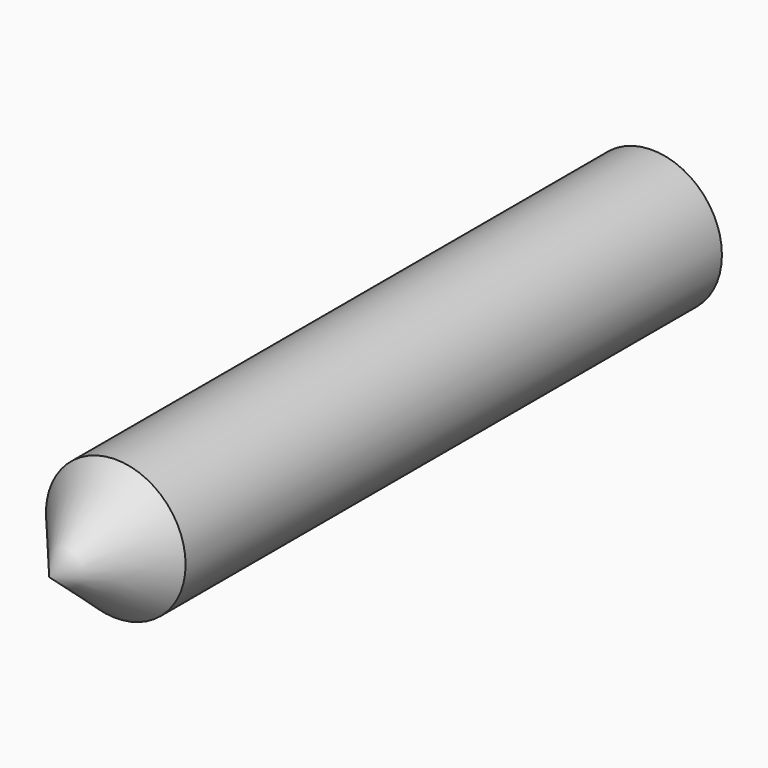
from build123d import *

# Parameters (mm, degrees)
F0_R     = 15.875
F0_R_2   = 12.7
F1_DEPTH = 152.4
F2_R     = 15.875


# Not quite as in the source:
# - an extrude whose draft closes it to a point is written as a loft to that point


with BuildPart() as f1:
    # F0 (on Front) → F1 (new body)
    with BuildSketch(Plane.XZ):
        Circle(F0_R)
        Circle(F0_R_2, mode=Mode.SUBTRACT)
    extrude(amount=F1_DEPTH)

    # F2 (on face) → F3 section 0
    with BuildSketch(Plane.XZ.offset(152.4), mode=Mode.PRIVATE) as f3_s0:
        Circle(F2_R)
    loft([f3_s0.sketch, Vertex(0, -171.3190882824, 0)], ruled=True)


solid = f1.part
